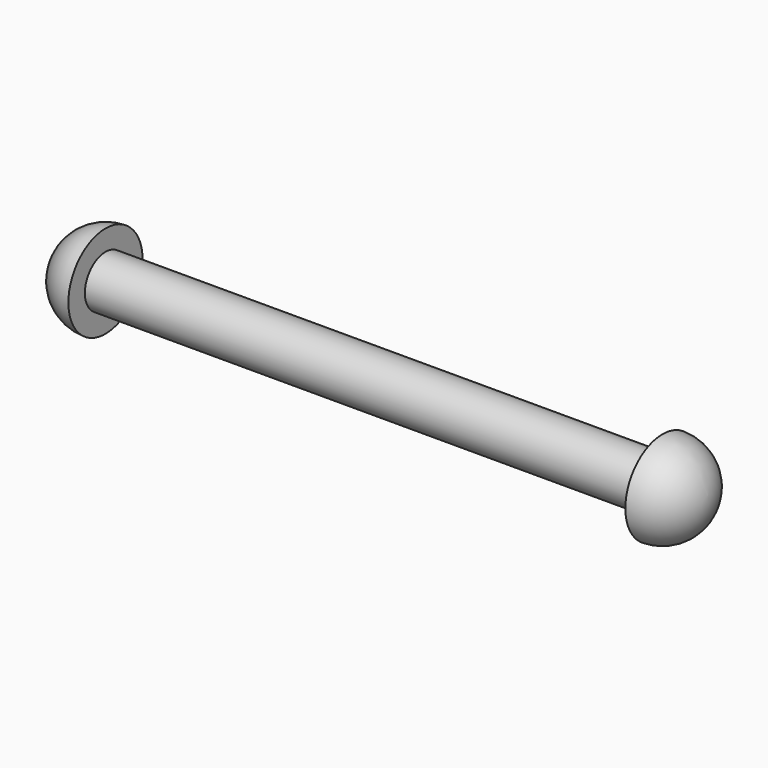
from build123d import *

# Parameters (mm, degrees)
F0_R     = 3.175
F1_DEPTH = 34.29


# Not quite as in the source:
# - a length typed as a fraction of an inch, garbled in the dataset ("3 / 203.2 mm" for 3/8 in), is restored
# - a feature names something its author has since deleted; it is built from what else it names


with BuildPart() as f1:
    # F0 (on Right) → F1 (new body)
    with BuildSketch(Plane.YZ):
        Circle(F0_R)
    extrude(amount=-F1_DEPTH)

    # F2 (on Front) → F3 (revolve)
    with BuildSketch(Plane.XZ):
        with BuildLine():
            Line((0, 3.175), (0, 0))
            Line((0, 0), (5.715, 0))
            ThreePointArc((5.715, 0), (4.0411152545, 4.0411152545), (0, 5.715))
            Line((0, 5.715), (0, 3.175))
        make_face()
    revolve(axis=Axis((0, 0, 0), (1, 0, 0)))

    # F4: F1 across face


with BuildPart() as f1_1:
    add(f1.part)
    add(f1.part.mirror(Plane(origin=(-34.29, 0, 0), x_dir=(0, 1, 0), z_dir=(-1, 0, 0))))


solid = f1_1.part
